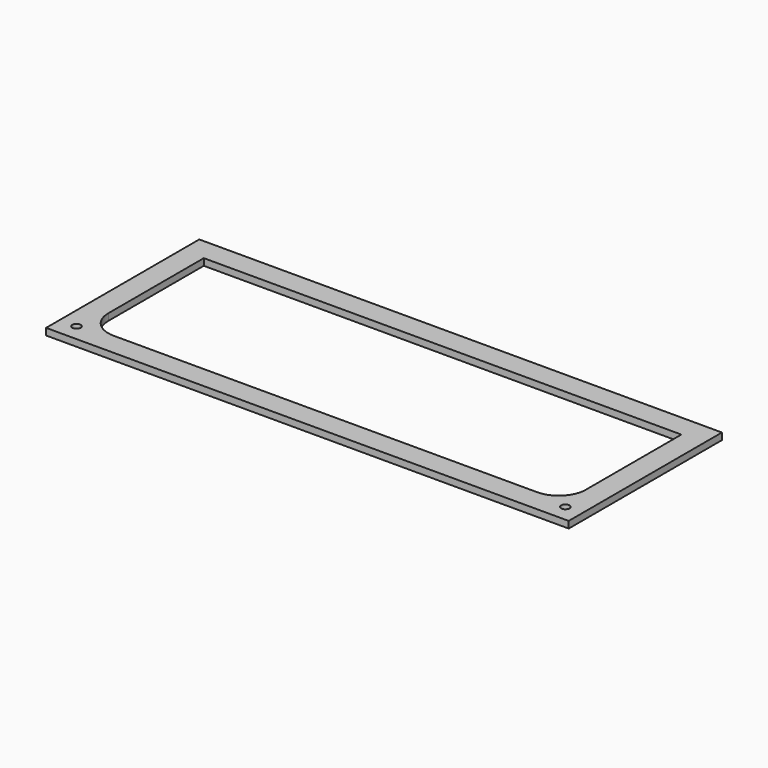
from build123d import *

# Parameters (mm, degrees)
F0_W     = 232
F0_H     = 85
F2_DEPTH = 3
F3_W     = 212
F3_H     = 65
F4_DEPTH = 3
F5_R     = 12
F6_R     = 1.85
F7_DEPTH = 3


# Not quite as in the source:
# - a feature names something its author has since deleted; it is built from what else it names


with BuildPart() as f2:
    # F0 (on Top) → F2 (new body)
    with BuildSketch(Plane.XY):
        Rectangle(F0_W, F0_H)
    extrude(amount=F2_DEPTH)

    # F3 (on face) → F4 (cut)
    with BuildSketch(Plane.XY.offset(3)):
        Rectangle(F3_W, F3_H)
    extrude(amount=-F4_DEPTH, mode=Mode.SUBTRACT)

    # F5
    f5_edges = [f2.edges().sort_by_distance(p)[0] for p in [
        (-106, -32.5, 1.5),
        (106, -32.5, 1.5),
    ]]
    fillet(f5_edges, radius=F5_R)

    # F6 (on face) → F7 (cut)
    with BuildSketch(Plane.XY.offset(3)):
        with Locations((-108.5, -35)):
            Circle(F6_R)
        with Locations((108.5, -35)):
            Circle(F6_R)
    extrude(amount=-F7_DEPTH, mode=Mode.SUBTRACT)


solid = f2.part
